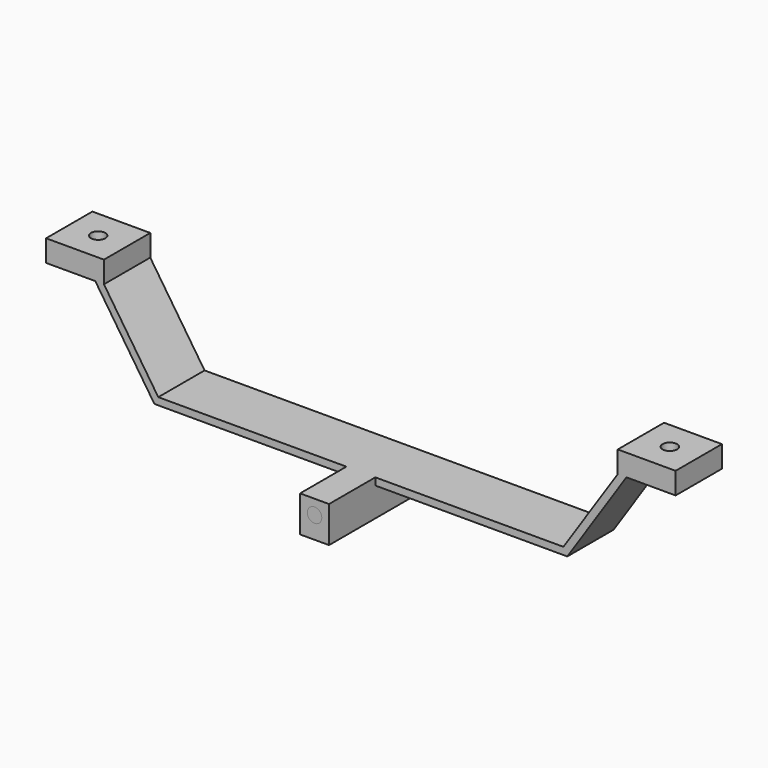
from build123d import *

# Parameters (mm, degrees)
F1_DEPTH = 12.7
F2_W     = 6.35
F2_H     = 12.7
F2_H_2   = 3.175
F3_DEPTH = 25.4
F4_R     = 3.175
F5_DEPTH = 25.4
F6_R     = 3.175
F7_DEPTH = 25.4
F8_R     = 3.175
F9_DEPTH = 25.4


# Not quite as in the source:
# - a feature names something its author has since deleted; it is built from what else it names


with BuildPart() as f1:
    # F0 (on Front) → F1 (new body, symmetric)
    with BuildSketch(Plane.XZ):
        Polygon((-110.9493968193, 35.8484322961), (-107.1362588495, 35.8484322961), (-107.1362588495, 45.3734322961), (-132.5362588495, 45.3734322961), (-132.5362588495, 35.8484322961), align=None)
        Polygon((94.5069370505, 0), (-83.2930629495, 0), (-107.1362588495, 35.8484322961), (-110.9493968193, 35.8484322961), (-109.7799148305, 34.090106941), (-84.9944726753, -3.175), (96.2083467763, -3.175), (122.1632709203, 35.8484322961), (118.3501329505, 35.8484322961), align=None)
        Polygon((118.3501329505, 45.3734322961), (118.3501329505, 35.8484322961), (122.1632709203, 35.8484322961), (128.4984556522, 45.3734322961), align=None)
        Polygon((128.4984556522, 45.3734322961), (122.1632709203, 35.8484322961), (143.7501329505, 35.8484322961), (143.7501329505, 45.3734322961), align=None)
    extrude(amount=F1_DEPTH, both=True)

    # F2 (on face) → F3 (join, symmetric)
    with BuildSketch(Plane.XZ.offset(12.7)):
        with Locations((2.4319370505, -9.525)):
            Rectangle(F2_W, F2_H)
        with Locations((8.7819370505, -9.525)):
            Rectangle(F2_W, F2_H)
        with Locations((8.7819370505, -1.5875)):
            Rectangle(F2_W, F2_H_2)
        Polygon((5.6069370505, -3.175), (5.6069370505, 0), (0, 0), (-0.7430629495, 0), (-0.7430629495, -3.175), align=None)
    extrude(amount=F3_DEPTH, both=True)

    # F6 (on face) → F7 (cut)
    with BuildSketch(Plane.XY.offset(45.3734322961)):
        with Locations((131.0501329505, 0)):
            Circle(F6_R)
    extrude(amount=-F7_DEPTH, mode=Mode.SUBTRACT)

    # F8 (on face) → F9 (cut)
    with BuildSketch(Plane.XY.offset(45.3734322961)):
        with Locations((-119.8362588495, 0)):
            Circle(F8_R)
    extrude(amount=-F9_DEPTH, mode=Mode.SUBTRACT)


with BuildPart() as f5:
    # F4 (on face) → F5 (new body)
    with BuildSketch(Plane.XZ.offset(38.1)):
        with Locations((5.6069370505, -6.35)):
            Circle(F4_R)
    extrude(amount=-F5_DEPTH)


solid = Compound([f1.part, f5.part])
